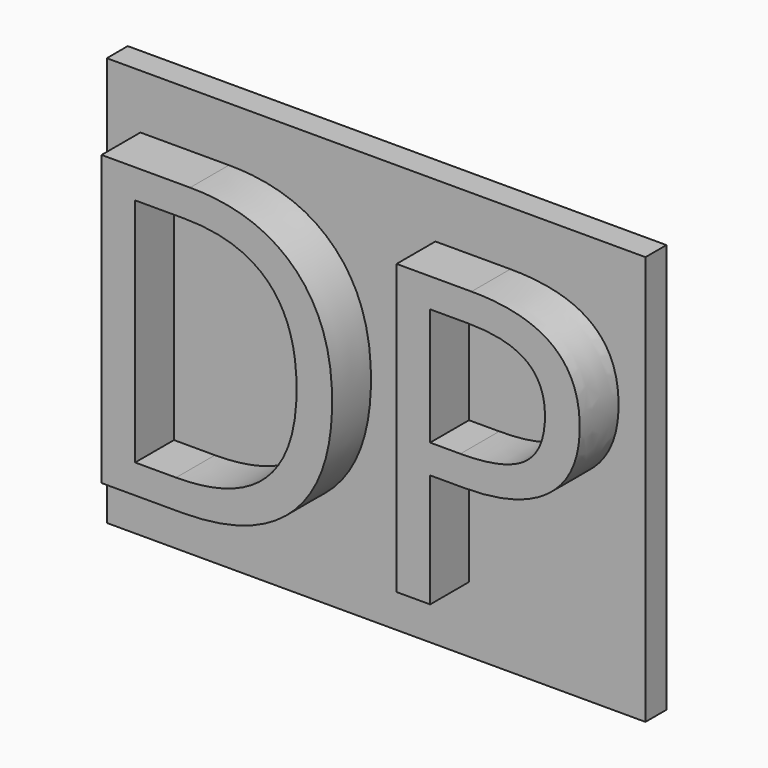
from build123d import *

# Parameters (mm, degrees)
F0_TEXT_SIZE = 105.8333333333
F1_DEPTH     = 12.7
F2_W         = 140.889339149
F2_H         = 107.0121340454
F3_DEPTH     = 6.858


# Not quite as in the source:
# - Text() gives the source's letters only with a copy of the font that has no kerning and outlines rounded to 1/6400 em; it was checked with that copy


with BuildPart() as f1:
    # F0 (on Front) → F1 (new body)
    with BuildSketch(Plane.XZ):
        with Locations((-47.6249968204, -39.1885698297)):
            Text('DP', F0_TEXT_SIZE, font='Open Sans', text_align=(TextAlign.LEFT, TextAlign.BOTTOM))
    extrude(amount=F1_DEPTH)

    # F2 (on Front) → F3 (join)
    with BuildSketch(Plane.XZ):
        with Locations((24.4115181267, -2.8895270079)):
            Rectangle(F2_W, F2_H)
    extrude(amount=-F3_DEPTH)


solid = f1.part
